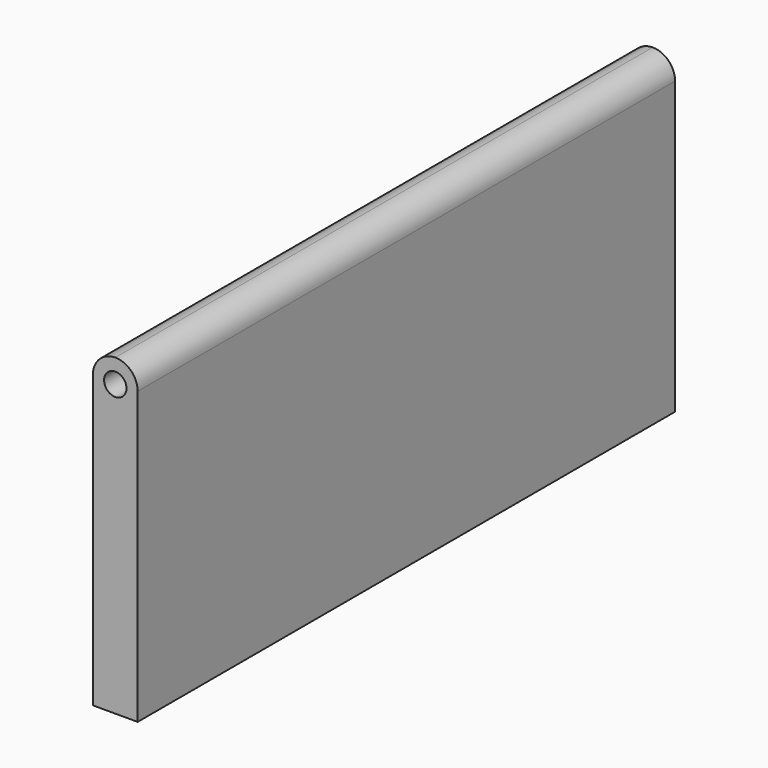
from build123d import *

# Parameters (mm, degrees)
F0_W     = 150
F0_H     = 70
F1_DEPTH = 10
F2_R     = 4.99999
F3_R     = 2.5
F4_DEPTH = 80.75
F5_T     = -1


# Not quite as in the source:
# - a fillet or chamfer is up to 0.001 mm smaller than in the source, because OpenCascade refuses the exact size


with BuildPart() as f1:
    # F0 (on Right) → F1 (new body)
    with BuildSketch(Plane.YZ):
        Rectangle(F0_W, F0_H)
    extrude(amount=F1_DEPTH)

    # F2 (radius 5 in the source; OpenCascade refuses exactly that, so slightly less here)
    f2_edges = [f1.edges().sort_by_distance(p)[0] for p in [
        (10, 0, 35),
        (0, 0, 35),
    ]]
    fillet(f2_edges, radius=F2_R)

    # F3 (on Front) → F4 (cut, symmetric)
    with BuildSketch(Plane.XZ):
        with Locations((5, 29.747851193)):
            Circle(F3_R)
    extrude(amount=F4_DEPTH, both=True, mode=Mode.SUBTRACT)

    # F5
    f5_openings = [f1.faces().sort_by_distance(p)[0] for p in [
        (5, 0, -35),
    ]]
    offset(amount=F5_T, openings=f5_openings)


solid = f1.part
